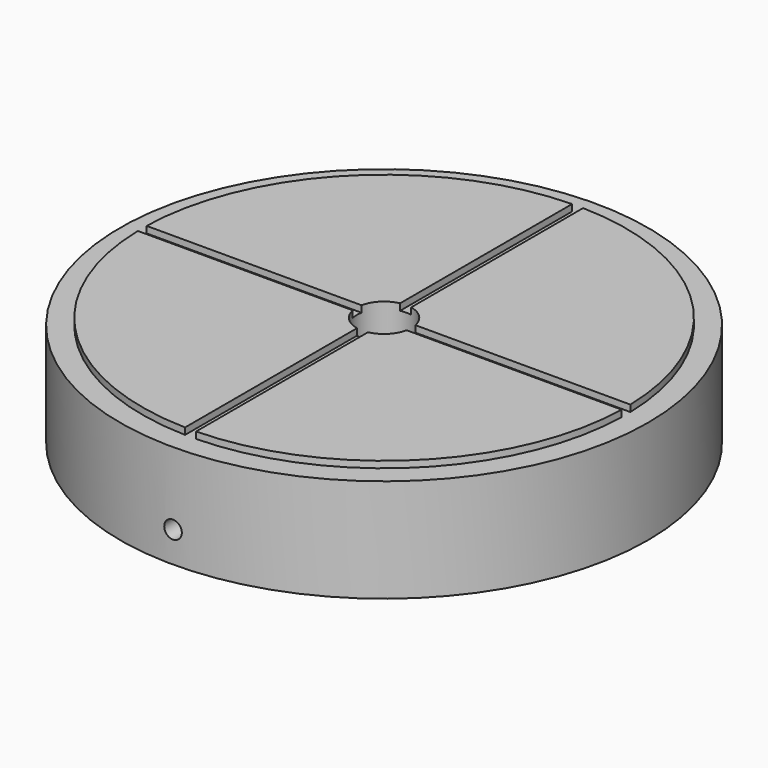
from build123d import *

# Parameters (mm, degrees)
F0_R          = 120
F1_DEPTH      = 12
F1_DEPTH_BACK = 38
F2_R          = 110
F2_R_2        = 17.5
F3_DEPTH      = 38
F4_R          = 5
F5_R          = 15.2795
F6_DEPTH      = 15.2795
F8_R          = 120
F9_DEPTH      = 5
F10_R         = 12.5
F11_DEPTH     = 55.001
F12_R         = 120
F12_R_2       = 110
F13_DEPTH     = 3
F14_W         = 5
F14_H         = 122.5
F14_W_2       = 122.5
F14_H_2       = 5
F15_DEPTH     = 3
F16_R         = 136.7884680592
F16_R_2       = 100.9393969777
F17_DEPTH     = 5
F19_R         = 4
F20_DEPTH     = 25
F22_R         = 4
F23_DEPTH     = 25


# Not quite as in the source:
# - a fillet or chamfer that OpenCascade refuses, or shapes differently, is made with other operations: its cross-section is extruded or revolved along the edge and cut away or added


with BuildPart() as f1:
    # F0 (on Top) → F1 (new body, two sides)
    with BuildSketch(Plane.XY) as f1_sk:
        Circle(F0_R)
    extrude(amount=F1_DEPTH)
    extrude(f1_sk.sketch, amount=-F1_DEPTH_BACK)

    # F2 (on face) → F3 (cut)
    with BuildSketch(Plane(origin=(0, 0, -38), x_dir=(1, 0, 0), z_dir=(0, 0, -1))):
        Circle(F2_R)
        Circle(F2_R_2, mode=Mode.SUBTRACT)
    extrude(amount=-F3_DEPTH, mode=Mode.SUBTRACT)

    # F4
    f4_edges = [f1.edges().sort_by_distance(p)[0] for p in [
        (-17.5, 0, 0),
        (-110, 0, 0),
    ]]
    fillet(f4_edges, radius=F4_R)

    # F5 (on face) → F6 (cut)
    with BuildSketch(Plane(origin=(0, 0, 0), x_dir=(1, 0, 0), z_dir=(0, 0, -1))):
        with Locations((-60, 60)):
            Circle(F5_R)
        with Locations((-60, -60)):
            Circle(F5_R)
        with Locations((60, -60)):
            Circle(F5_R)
        with Locations((60, 60)):
            Circle(F5_R)
    extrude(amount=-F6_DEPTH, mode=Mode.SUBTRACT)

    # F8 (on face) → F9 (join)
    with BuildSketch(Plane.XY.offset(12)):
        Circle(F8_R)
    extrude(amount=F9_DEPTH)

    # F10 (on face) → F11 (cut, through all)
    with BuildSketch(Plane(origin=(0, 0, -38), x_dir=(1, 0, 0), z_dir=(0, 0, -1))):
        Circle(F10_R)
    extrude(amount=-F11_DEPTH, mode=Mode.SUBTRACT)

    # F12 (on face) → F13 (cut)
    with BuildSketch(Plane.XY.offset(17)):
        Circle(F12_R)
        Circle(F12_R_2, mode=Mode.SUBTRACT)
    extrude(amount=-F13_DEPTH, mode=Mode.SUBTRACT)

    # F14 (on face) → F15 (cut)
    with BuildSketch(Plane.XY.offset(17)):
        with Locations((0, -63.75)):
            Rectangle(F14_W, F14_H)
        with Locations((-63.75, 0)):
            Rectangle(F14_W_2, F14_H_2)
        Rectangle(F14_W, F14_H_2)
        with Locations((63.75, 0)):
            Rectangle(F14_W_2, F14_H_2)
        with Locations((0, 63.75)):
            Rectangle(F14_W, F14_H)
    extrude(amount=-F15_DEPTH, mode=Mode.SUBTRACT)

    # F16 (on face) → F17 (cut)
    with BuildSketch(Plane(origin=(0, 0, -38), x_dir=(1, 0, 0), z_dir=(0, 0, -1))):
        Circle(F16_R)
        Circle(F16_R_2, mode=Mode.SUBTRACT)
    extrude(amount=-F17_DEPTH, mode=Mode.SUBTRACT)

    # F18: fillet of radius 15.2795 on 4 edges, made by hand

    # F18_s1 → F18_t2 (revolve)
    with BuildSketch(Plane.XZ.offset(60)):
        with BuildLine():
            ThreePointArc((75.2795, 0), (69.9309062658, 8.6278977111), (60.3560955627, 12))
            Line((60.3560955627, 12), (75.2795, 12))
            Line((75.2795, 12), (75.2795, 0))
        make_face()
    revolve(axis=Axis((60, -60, 12), (0, 0, -1)))

    # F18_s3 → F18_t4 (revolve)
    with BuildSketch(Plane.XZ.offset(60)):
        with BuildLine():
            ThreePointArc((-44.7205, 0), (-50.0690937342, 8.6278977111), (-59.6439044373, 12))
            Line((-59.6439044373, 12), (-44.7205, 12))
            Line((-44.7205, 12), (-44.7205, 0))
        make_face()
    revolve(axis=Axis((-60, -60, 12), (0, 0, -1)))

    # F18_s5 → F18_t6 (revolve)
    with BuildSketch(Plane.XZ.offset(-60)):
        with BuildLine():
            ThreePointArc((-44.7205, 0), (-50.0690937342, 8.6278977111), (-59.6439044373, 12))
            Line((-59.6439044373, 12), (-44.7205, 12))
            Line((-44.7205, 12), (-44.7205, 0))
        make_face()
    revolve(axis=Axis((-60, 60, 12), (0, 0, -1)))

    # F18_s7 → F18_t8 (revolve)
    with BuildSketch(Plane.XZ.offset(-60)):
        with BuildLine():
            ThreePointArc((75.2795, 0), (69.9309062658, 8.6278977111), (60.3560955627, 12))
            Line((60.3560955627, 12), (75.2795, 12))
            Line((75.2795, 12), (75.2795, 0))
        make_face()
    revolve(axis=Axis((60, 60, 12), (0, 0, -1)))

    # F19 (on offset) → F20 (cut)
    with BuildSketch(Plane.XZ.offset(120)):
        with Locations((0, -19)):
            Circle(F19_R)
    extrude(amount=-F20_DEPTH, mode=Mode.SUBTRACT)

    # F22 (on offset) → F23 (cut)
    with BuildSketch(Plane.XZ.offset(-120)):
        with Locations((0, -19)):
            Circle(F22_R)
    extrude(amount=F23_DEPTH, mode=Mode.SUBTRACT)


solid = f1.part
